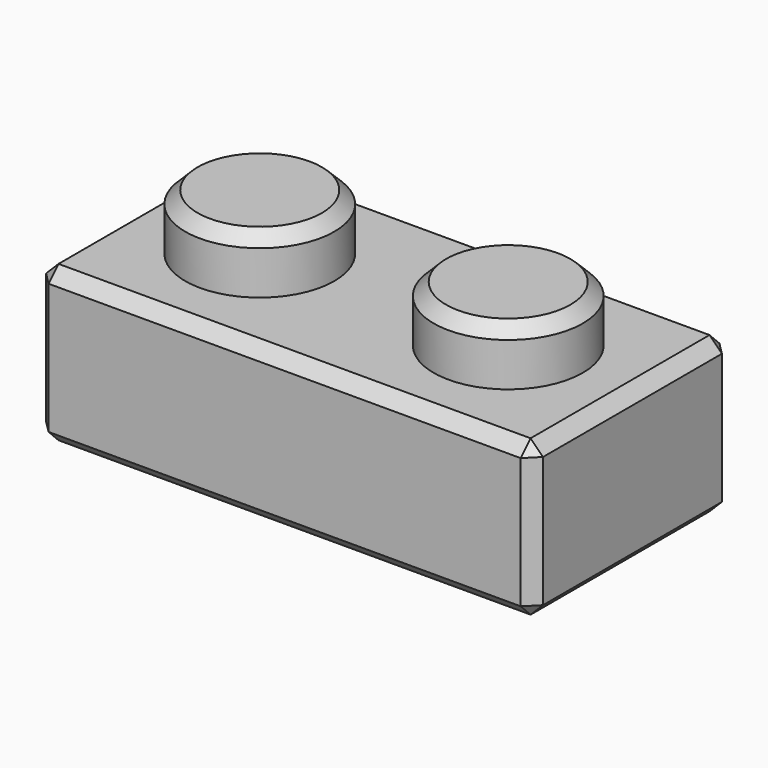
from build123d import *

# Parameters (mm, degrees)
F0_W     = 16
F0_H     = 8
F0_W_2   = 14
F0_H_2   = 6
F0_R     = 2.995
F0_R_2   = 2.55
F0_R_3   = 2.4
F1_DEPTH = 1
F2_DEPTH = 1.8
F3_DEPTH = 5
F4_SIZE  = 0.4


# Not quite as in the source:
# - a feature names something its author has since deleted; it is built from what else it names


with BuildPart() as f1:
    # F0 (on Top) → F1 (new body)
    with BuildSketch(Plane.XY):
        Rectangle(F0_W, F0_H)
        Rectangle(F0_W_2, F0_H_2, mode=Mode.SUBTRACT)
        Rectangle(F0_W_2, F0_H_2)
        with Locations((-4, 0)):
            Circle(F0_R, mode=Mode.SUBTRACT)
        with Locations((4, 0)):
            Circle(F0_R, mode=Mode.SUBTRACT)
        with Locations((-4, 0)):
            Circle(F0_R)
        with Locations((-4, 0)):
            Circle(F0_R_2, mode=Mode.SUBTRACT)
        with Locations((4, 0)):
            Circle(F0_R)
        with Locations((4, 0)):
            Circle(F0_R_2, mode=Mode.SUBTRACT)
        with Locations((-4, 0)):
            Circle(F0_R_2)
        with Locations((-4, 0)):
            Circle(F0_R_3, mode=Mode.SUBTRACT)
        with Locations((4, 0)):
            Circle(F0_R_2)
        with Locations((4, 0)):
            Circle(F0_R_3, mode=Mode.SUBTRACT)
        with Locations((4, 0)):
            Circle(F0_R_3)
        with Locations((-4, 0)):
            Circle(F0_R_3)
    extrude(amount=-F1_DEPTH)

    # F0 (on Top) → F2 (join)
    with BuildSketch(Plane.XY):
        with Locations((-4, 0)):
            Circle(F0_R_3)
        with Locations((4, 0)):
            Circle(F0_R_3)
    extrude(amount=F2_DEPTH)

    # F0 (on Top) → F3 (join)
    with BuildSketch(Plane.XY):
        Rectangle(F0_W, F0_H)
        Rectangle(F0_W_2, F0_H_2, mode=Mode.SUBTRACT)
        Rectangle(F0_W_2, F0_H_2)
        with Locations((-4, 0)):
            Circle(F0_R, mode=Mode.SUBTRACT)
        with Locations((4, 0)):
            Circle(F0_R, mode=Mode.SUBTRACT)
        with Locations((4, 0)):
            Circle(F0_R)
        with Locations((4, 0)):
            Circle(F0_R_2, mode=Mode.SUBTRACT)
        with Locations((-4, 0)):
            Circle(F0_R)
        with Locations((-4, 0)):
            Circle(F0_R_2, mode=Mode.SUBTRACT)
    extrude(amount=-F3_DEPTH)

    # F4
    f4_edges = [f1.edges().sort_by_distance(p)[0] for p in [
        (-6.4, 0, 1.8),
        (1.6, 0, 1.8),
        (-8, -4, -2.5),
        (0, -4, -5),
        (8, -4, -2.5),
        (0, -4, 0),
        (-8, 4, -2.5),
        (-8, 0, -5),
        (-8, 0, 0),
        (8, 4, -2.5),
        (0, 4, -5),
        (0, 4, 0),
        (8, 0, -5),
        (8, 0, 0),
        (1.45, 0, -5),
        (-6.55, 0, -5),
    ]]
    chamfer(f4_edges, length=F4_SIZE)


solid = f1.part
